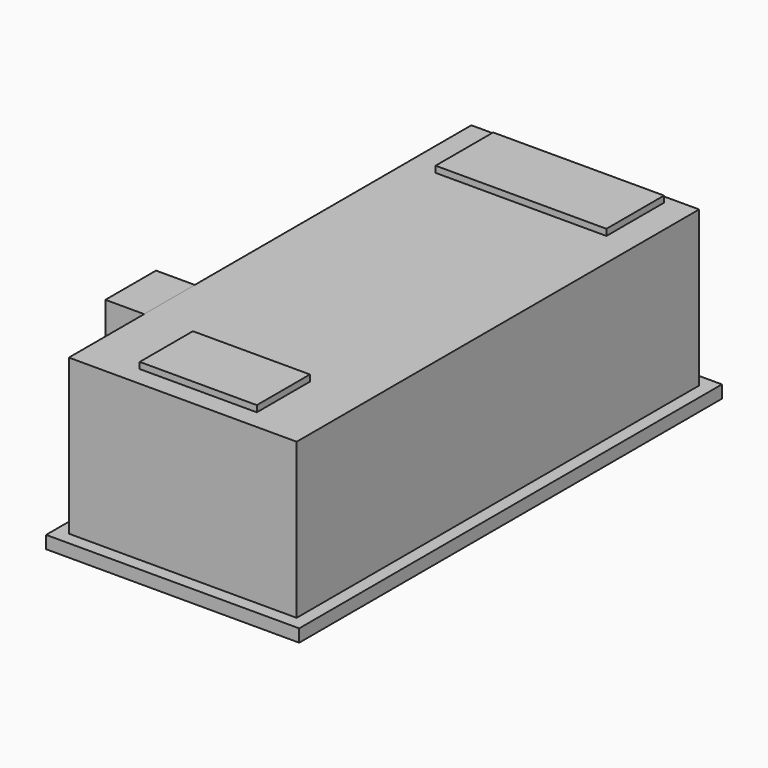
from build123d import *

# Parameters (mm, degrees)
F0_W         = 1828.8
F0_H         = 1244.6
F1_DEPTH     = 4038.6
F2_W         = 939.8
F2_H         = 533.4
F3_DEPTH     = 50.8
F4_W         = 2032
F4_H         = 101.6
F5_DEPTH     = 4140.2
F6_DEPTH     = 101.6
F7_W         = 508
F7_H         = 762
F8_DEPTH     = 311.15
F9_TEXT_SIZE = 388.0555555556
F10_DEPTH    = 25.4
F11_W        = 1371.6
F11_H        = 577.85
F12_DEPTH    = 50.8
F13_W        = 1371.6
F13_H        = 577.85
F14_DEPTH    = 50.8


# Not quite as in the source:
# - Text() gives the source's letters only with a copy of the font that has no kerning and outlines rounded to 1/6400 em; it was checked with that copy


with BuildPart() as f1:
    # F0 (on Front) → F1 (new body)
    with BuildSketch(Plane.XZ):
        with Locations((274.4598696411, 69.8617820535)):
            Rectangle(F0_W, F0_H)
    extrude(amount=F1_DEPTH)

    # F2 (on face) → F3 (join)
    with BuildSketch(Plane.XY.offset(692.1617820535)):
        with Locations((274.4598696411, -3616.325)):
            Rectangle(F2_W, F2_H)
    extrude(amount=F3_DEPTH)

    # F9 (on face) → F10 (join)
    with BuildSketch(Plane(origin=(-639.9401303589, 0, 0), x_dir=(0, -1, 0), z_dir=(-1, 0, 0))):
        with Locations((60.3798998959, -485.0257645123)):
            Text('AHU-G-7/8', F9_TEXT_SIZE, font='Open Sans', text_align=(TextAlign.LEFT, TextAlign.BOTTOM))
    extrude(amount=F10_DEPTH)

    # F11 (on face) → F12 (join)
    with BuildSketch(Plane.XY.offset(692.1617820535)):
        with Locations((274.4598696411, -355.6)):
            Rectangle(F11_W, F11_H)
    extrude(amount=F12_DEPTH)

    # F13 (on face) → F14 (join)
    with BuildSketch(Plane(origin=(0, 0, 0), x_dir=(-1, 0, 0), z_dir=(0, 1, 0))):
        with Locations((-274.4598696411, 104.7867820535)):
            Rectangle(F13_W, F13_H)
    extrude(amount=F14_DEPTH)


with BuildPart() as f5:
    # F4 (on face) → F5 (new body)
    with BuildSketch(Plane.XZ.offset(4038.6)):
        with Locations((274.4598696411, -603.2382179465)):
            Rectangle(F4_W, F4_H)
    extrude(amount=-F5_DEPTH)

    # F6 (add): a face of the model
    f6_faces = [f5.faces().sort_by_distance(p)[0] for p in [
        (274.4598696411, -4038.6, -603.2382179465),
    ]]
    extrude(f6_faces, amount=F6_DEPTH)


with BuildPart() as f8:
    # F7 (on face) → F8 (new body)
    with BuildSketch(Plane(origin=(-639.9401303589, 0, 0), x_dir=(0, -1, 0), z_dir=(-1, 0, 0))):
        with Locations((3028.95, 311.1617820535)):
            Rectangle(F7_W, F7_H)
    extrude(amount=F8_DEPTH)


solid = Compound([f1.part, f5.part, f8.part])
